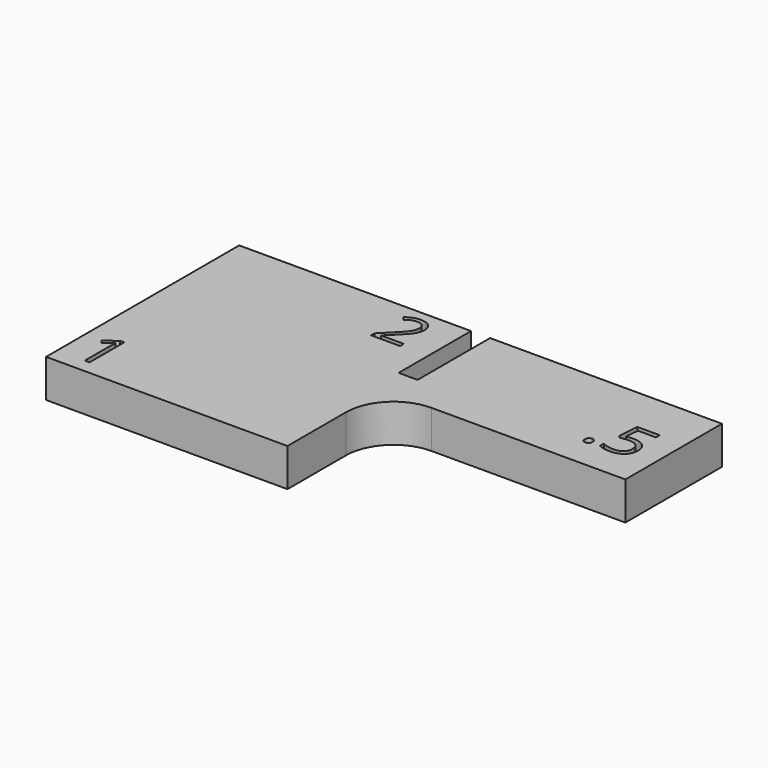
from build123d import *

# Parameters (mm, degrees)
F1_DEPTH       = 4
F2_W           = 2
F2_H           = 19.05
F3_DEPTH       = 2
F4_TEXT_SIZE   = 6.6277642165
F4_TEXT_SIZE_2 = 6.5050275427
F4_TEXT_SIZE_3 = 6.3822908689
F5_DEPTH       = 1


# Not quite as in the source:
# - Text() gives the source's letters only with a copy of the font that has no kerning and outlines rounded to 1/6400 em; it was checked with that copy


with BuildPart() as f1:
    # F0 (on Top) → F1 (new body)
    with BuildSketch(Plane.XY):
        with BuildLine():
            Line((-12.7, 12.7), (-12.7, -12.7))
            Line((-12.7, -12.7), (12.7, -12.7))
            Line((12.7, -12.7), (12.7, -5))
            ThreePointArc((12.7, -5), (14.1644660941, -1.4644660941), (17.7, 0))
            Line((17.7, 0), (38.1, 0))
            Line((38.1, 0), (38.1, 12.7))
            Line((38.1, 12.7), (-12.7, 12.7))
        make_face()
    extrude(amount=F1_DEPTH)

    # F2 (on face) → F3 (cut)
    with BuildSketch(Plane.XY.offset(4)):
        with Locations((12.7000364751, 12.6999945655)):
            Rectangle(F2_W, F2_H)
    extrude(amount=-F3_DEPTH, mode=Mode.SUBTRACT)

    # F4 (on face) → F5 (cut)
    with BuildSketch(Plane.XY.offset(4)):
        with Locations((30.5421613157, 3.1771266367)):
            Text('.5', F4_TEXT_SIZE, font='Open Sans', text_align=(TextAlign.LEFT, TextAlign.BOTTOM))
        with Locations((5.4450249299, 6.9770445116)):
            Text('2', F4_TEXT_SIZE_2, font='Open Sans', text_align=(TextAlign.LEFT, TextAlign.BOTTOM))
        with Locations((-11.5220518783, -11.2272137776)):
            Text('1', F4_TEXT_SIZE_3, font='Open Sans', text_align=(TextAlign.LEFT, TextAlign.BOTTOM))
    extrude(amount=-F5_DEPTH, mode=Mode.SUBTRACT)


solid = f1.part
